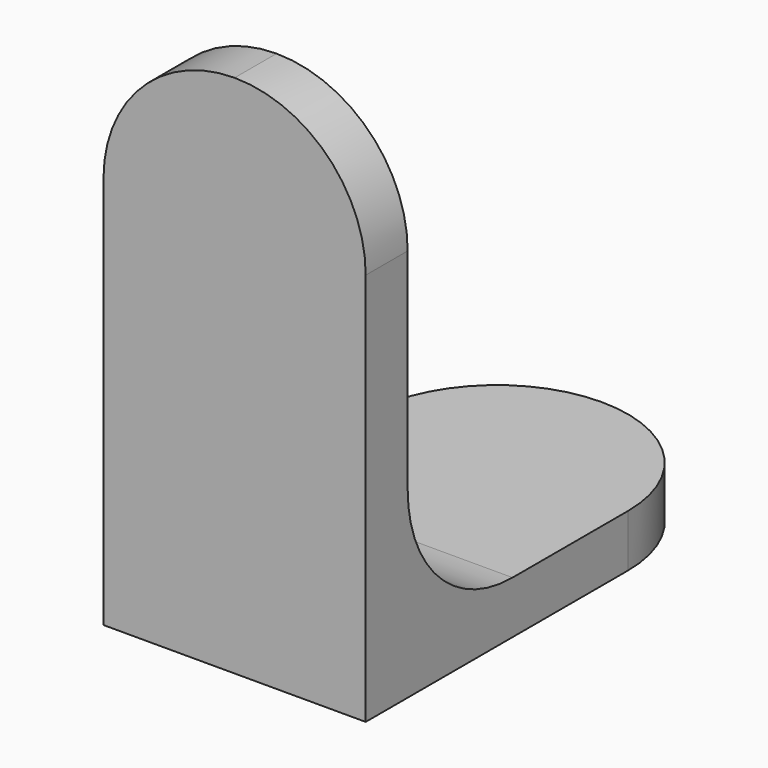
from build123d import *

# Parameters (mm, degrees)
F0_W     = 4
F0_H     = 4
F0_W_2   = 31
F0_H_2   = 36
F1_DEPTH = 10
F2_R     = 9.99999


# Not quite as in the source:
# - a fillet or chamfer is up to 0.001 mm smaller than in the source, because OpenCascade refuses the exact size


with BuildPart() as f1:
    # F0 (on Right) → F1 (new body, symmetric)
    with BuildSketch(Plane.YZ):
        with Locations((2, 2)):
            Rectangle(F0_W, F0_H)
        with Locations((19.5, 2)):
            Rectangle(F0_W_2, F0_H)
        with Locations((2, 22)):
            Rectangle(F0_W, F0_H_2)
    extrude(amount=F1_DEPTH, both=True)

    # F2 (radius 10 in the source; OpenCascade refuses exactly that, so slightly less here)
    f2_edges = [f1.edges().sort_by_distance(p)[0] for p in [
        (0, 4, 4),
        (10, 35, 2),
        (-10, 35, 2),
        (10, 2, 40),
        (-10, 2, 40),
    ]]
    fillet(f2_edges, radius=F2_R)


solid = f1.part
